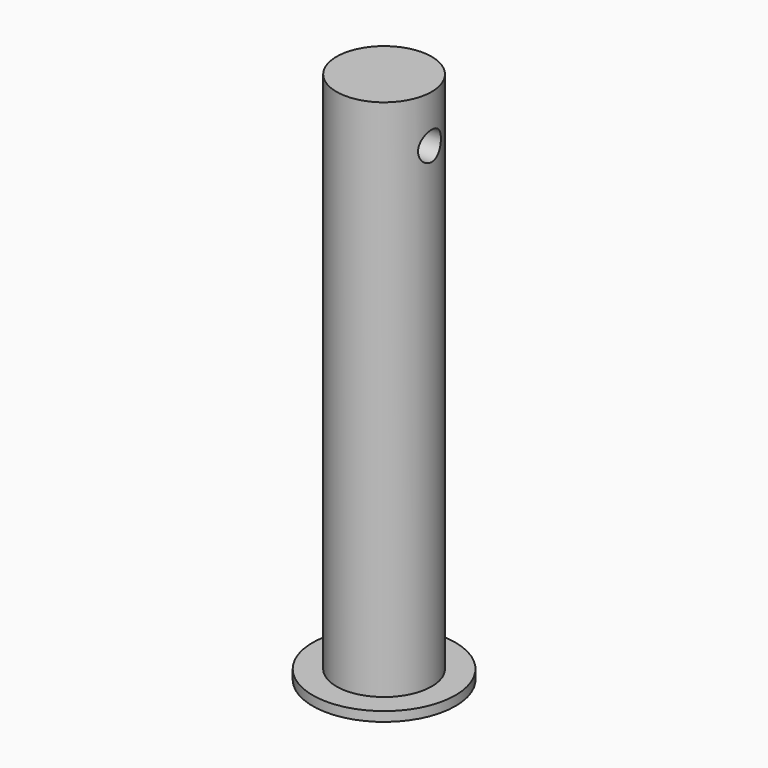
from build123d import *

# Parameters (mm, degrees)
F0_R     = 7.5
F1_DEPTH = 1
F2_R     = 5
F3_DEPTH = 55
F5_R     = 1.5
F6_DEPTH = 32.501
F7_DEPTH = 48


with BuildPart() as f1:
    # F0 (on Top) → F1 (new body)
    with BuildSketch(Plane.XY):
        Circle(F0_R)
    extrude(amount=F1_DEPTH)

    # F2 (on face) → F3 (join)
    with BuildSketch(Plane.XY.offset(1)):
        Circle(F2_R)
    extrude(amount=F3_DEPTH)

    # F5 (on face) → F6 (cut, through all)
    with BuildSketch(Plane.YZ.offset(25)):
        with Locations((0, 51)):
            Circle(F5_R)
    extrude(amount=-F6_DEPTH, mode=Mode.SUBTRACT)

    # F2 (on face) → F7 (join)
    with BuildSketch(Plane.XY.offset(1)):
        Circle(F2_R)
    extrude(amount=F7_DEPTH)


solid = f1.part
